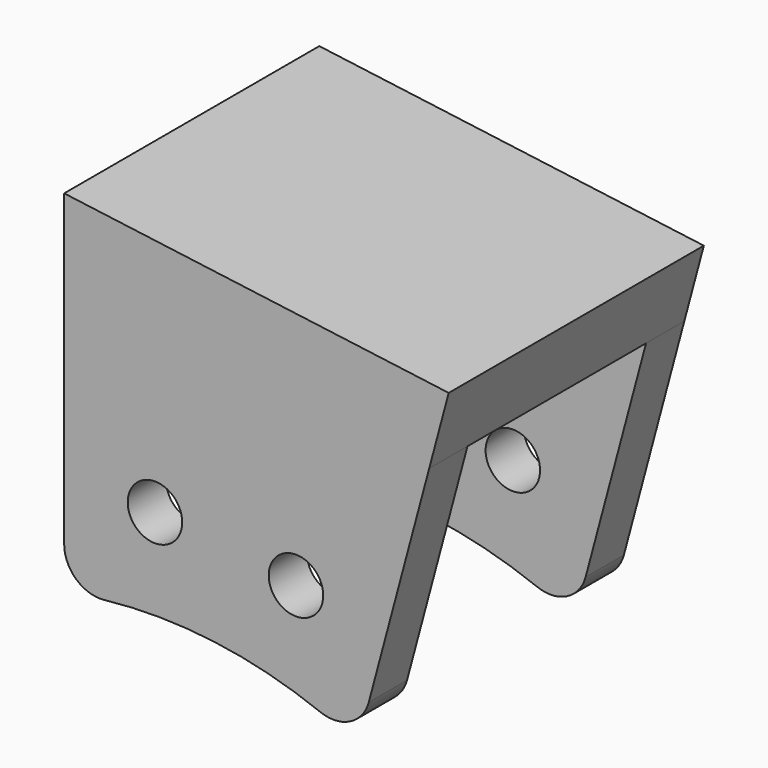
from build123d import *

# Parameters (mm, degrees)
F0_R     = 1.2813159657
F1_DEPTH = 7.5
F2_DEPTH = 5.25


# Not quite as in the source:
# - ends of sketch curves that miss each other by under 0.0002 mm in the source are joined


with BuildPart() as f1:
    # F0 (on Front) → F1 (new body, symmetric)
    with BuildSketch(Plane.XZ):
        with BuildLine():
            ThreePointArc((7.8928847665, 2.2551549829), (-0.5468394213, 4.4913902739), (-9.2777672646, 4.515713911))
            Line((-9.2777672646, 4.515713911), (-9.27776646, -6.4638420574))
            ThreePointArc((-9.27776646, -6.4638420574), (-8.7082936227, -7.7372240383), (-7.3795216285, -8.1616848044))
            ThreePointArc((-7.3795216285, -8.1616848044), (-2.2192897787, -8.212150504), (2.7781677389, -9.4989699664))
            ThreePointArc((2.7781677389, -9.4989699664), (4.1715212346, -9.432884372), (5.0511658084, -8.3502824825))
            Line((5.0511658084, -8.3502824825), (7.8928847665, 2.2551549829))
        make_face()
        with Locations((-5.0067132411, -3.7583980654)):
            Circle(F0_R, mode=Mode.SUBTRACT)
        with Locations((1.6258659514, -4.6315961033)):
            Circle(F0_R, mode=Mode.SUBTRACT)
        with BuildLine():
            Line((8.8106123745, 5.6801667894), (-9.27776646, 8.0615492201))
            Line((-9.27776646, 8.0615492201), (-9.27776646, 4.515713911))
            ThreePointArc((-9.27776646, 4.515713911), (-0.5468394213, 4.4913902739), (7.8928847665, 2.2551549829))
            Line((7.8928847665, 2.2551549829), (8.8106123745, 5.6801667894))
        make_face()
    extrude(amount=F1_DEPTH, both=True)

    # F0 (on Front) → F2 (cut, symmetric)
    with BuildSketch(Plane.XZ):
        with BuildLine():
            ThreePointArc((7.8928847665, 2.2551549829), (-0.5468394213, 4.4913902739), (-9.2777672646, 4.515713911))
            Line((-9.2777672646, 4.515713911), (-9.27776646, -6.4638420574))
            ThreePointArc((-9.27776646, -6.4638420574), (-8.7082936227, -7.7372240383), (-7.3795216285, -8.1616848044))
            ThreePointArc((-7.3795216285, -8.1616848044), (-2.2192897787, -8.212150504), (2.7781677389, -9.4989699664))
            ThreePointArc((2.7781677389, -9.4989699664), (4.1715212346, -9.432884372), (5.0511658084, -8.3502824825))
            Line((5.0511658084, -8.3502824825), (7.8928847665, 2.2551549829))
        make_face()
        with Locations((-5.0067132411, -3.7583980654)):
            Circle(F0_R, mode=Mode.SUBTRACT)
        with Locations((1.6258659514, -4.6315961033)):
            Circle(F0_R, mode=Mode.SUBTRACT)
        with Locations((-5.0067132411, -3.7583980654)):
            Circle(F0_R)
        with Locations((1.6258659514, -4.6315961033)):
            Circle(F0_R)
    extrude(amount=F2_DEPTH, both=True, mode=Mode.SUBTRACT)


solid = f1.part
